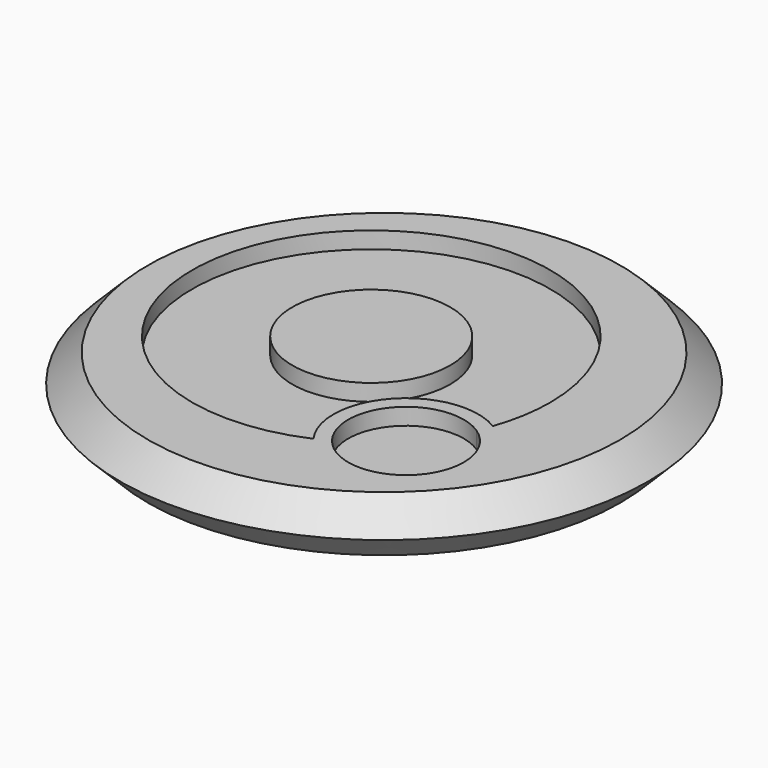
from build123d import *

# Parameters (mm, degrees)
F0_R     = 9.5
F1_DEPTH = 2
F2_SIZE  = 0.99999
F3_R     = 2.8417127556
F4_DEPTH = 0.6


# Not quite as in the source:
# - a fillet or chamfer is up to 0.001 mm smaller than in the source, because OpenCascade refuses the exact size


with BuildPart() as f1:
    # F0 (on Top) → F1 (new body)
    with BuildSketch(Plane.XY):
        Circle(F0_R)
    extrude(amount=F1_DEPTH)

    # F2 (size 1 in the source; OpenCascade refuses exactly that, so slightly less here)
    f2_edges = [f1.edges().sort_by_distance(p)[0] for p in [
        (-9.5, 0, 2),
        (-9.5, 0, 0),
    ]]
    chamfer(f2_edges, length=F2_SIZE)

    # F3 (on face) → F4 (cut)
    with BuildSketch(Plane.XY.offset(2)):
        with BuildLine():
            ThreePointArc((5.185311865, -1.585620522), (5.4568534532, -0.5346363532), (5.5482306838, 0.5470071919))
            ThreePointArc((5.5482306838, 0.5470071919), (-6.3080923619, 4.0561385788), (1.7284324719, -5.3407049258))
            ThreePointArc((1.7284324719, -5.3407049258), (1.9271777373, -2.0549469321), (5.185311865, -1.585620522))
        make_face()
        with Locations((-0.8992319345, 0.5470071919)):
            Circle(F3_R, mode=Mode.SUBTRACT)
        with BuildLine():
            ThreePointArc((4.9880163164, -2.0816963378), (2.3134948891, -2.4105852235), (2.2065269261, -5.1031287457))
            ThreePointArc((2.2065269261, -5.1031287457), (3.8442696915, -3.8197955903), (4.9880163164, -2.0816963378))
        make_face()
        with BuildLine():
            ThreePointArc((4.9880163164, -2.0816963378), (3.8442696915, -3.8197955903), (2.2065269261, -5.1031287457))
            ThreePointArc((2.2065269261, -5.1031287457), (4.5230773814, -5.7866116654), (5.9249295276, -3.8197955903))
            ThreePointArc((5.9249295276, -3.8197955903), (5.6757845042, -2.8325272153), (4.9880163164, -2.0816963378))
        make_face()
    extrude(amount=-F4_DEPTH, mode=Mode.SUBTRACT)


solid = f1.part
